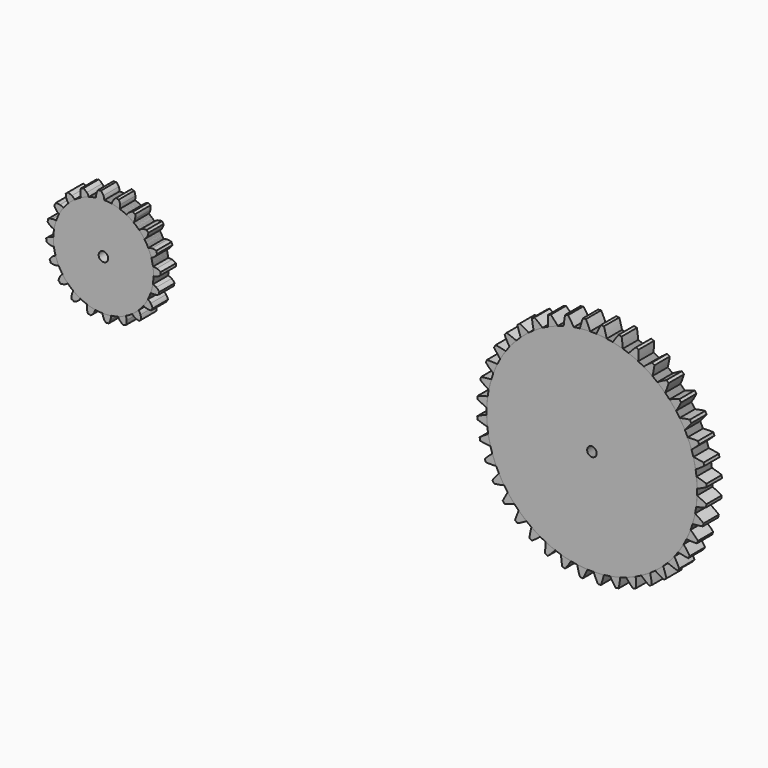
from build123d import *

# Parameters (mm, degrees)
F1_DEPTH = 25.4
F2_COUNT = 20
F4_D     = 12.7
F4_2_D   = 12.7
F4_3_D   = 12.7
F4_4_D   = 12.7
F4_5_D   = 12.7
F4_6_D   = 12.7
F4_7_D   = 12.7
F4_8_D   = 12.7
F4_9_D   = 12.7
F4_10_D  = 12.7
F4_11_D  = 12.7
F4_12_D  = 12.7
F4_13_D  = 12.7
F4_14_D  = 12.7
F4_15_D  = 12.7
F4_16_D  = 12.7
F4_17_D  = 12.7
F4_18_D  = 12.7
F4_19_D  = 12.7
F4_20_D  = 12.7
F5_R     = 6.35
F6_DEPTH = 25.4
F7_COUNT = 40


with BuildPart() as f1:
    # F0 (on Front) → F1 (new body)
    with BuildSketch(Plane.XZ):
        with BuildLine():
            ThreePointArc((-9.7867536931, 65.6960325526), (-43.3687864365, -50.3080272325), (66.421, 0))
            ThreePointArc((66.421, 0), (47.3638595406, 46.5662329421), (1.1279736855, 66.4114215807))
            ThreePointArc((1.1279736855, 66.4114215807), (-4.3441412466, 66.2787875404), (-9.7867536931, 65.6960325526))
        make_face()
        with BuildLine():
            ThreePointArc((-9.7867536931, 65.6960325526), (-4.3441412466, 66.2787875404), (1.1279736855, 66.4114215807))
            ThreePointArc((1.1279736855, 66.4114215807), (0.8169736788, 68.9502136588), (0, 71.374))
            ThreePointArc((0, 71.374), (-1.4134778135, 73.8905086139), (-3.2325792895, 76.1314023983))
            ThreePointArc((-3.2325792895, 76.1314023983), (-4.9594819457, 75.6670723933), (-6.7322179379, 75.9020239627))
            ThreePointArc((-6.7322179379, 75.9020239627), (-8.2432614157, 73.4428609463), (-9.3161764435, 70.7633855357))
            ThreePointArc((-9.3161764435, 70.7633855357), (-9.8097931974, 68.2536985592), (-9.7867536931, 65.6960325526))
        make_face()
    extrude(amount=F1_DEPTH)


with BuildPart() as f2_1:
    # F2: instance of F1
    add(f1.part.rotate(Axis((0, 0, 0), (0, 1, 0)), 1 * 360 / F2_COUNT))

    # F4#2 (through all)
    with Locations(Plane.XZ.offset(25.4)):
        with Locations((0, 0)):
            Hole(F4_2_D / 2)


with BuildPart() as f2_2:
    # F2: instance of F1
    add(f1.part.rotate(Axis((0, 0, 0), (0, 1, 0)), 2 * 360 / F2_COUNT))

    # F4#3 (through all)
    with Locations(Plane.XZ.offset(25.4)):
        with Locations((0, 0)):
            Hole(F4_3_D / 2)


with BuildPart() as f2_3:
    # F2: instance of F1
    add(f1.part.rotate(Axis((0, 0, 0), (0, 1, 0)), 3 * 360 / F2_COUNT))

    # F4#4 (through all)
    with Locations(Plane.XZ.offset(25.4)):
        with Locations((0, 0)):
            Hole(F4_4_D / 2)


with BuildPart() as f2_4:
    # F2: instance of F1
    add(f1.part.rotate(Axis((0, 0, 0), (0, 1, 0)), 4 * 360 / F2_COUNT))

    # F4#5 (through all)
    with Locations(Plane.XZ.offset(25.4)):
        with Locations((0, 0)):
            Hole(F4_5_D / 2)


with BuildPart() as f2_5:
    # F2: instance of F1
    add(f1.part.rotate(Axis((0, 0, 0), (0, 1, 0)), 5 * 360 / F2_COUNT))

    # F4#6 (through all)
    with Locations(Plane.XZ.offset(25.4)):
        with Locations((0, 0)):
            Hole(F4_6_D / 2)


with BuildPart() as f2_6:
    # F2: instance of F1
    add(f1.part.rotate(Axis((0, 0, 0), (0, 1, 0)), 6 * 360 / F2_COUNT))

    # F4#7 (through all)
    with Locations(Plane.XZ.offset(25.4)):
        with Locations((0, 0)):
            Hole(F4_7_D / 2)


with BuildPart() as f2_7:
    # F2: instance of F1
    add(f1.part.rotate(Axis((0, 0, 0), (0, 1, 0)), 7 * 360 / F2_COUNT))

    # F4#8 (through all)
    with Locations(Plane.XZ.offset(25.4)):
        with Locations((0, 0)):
            Hole(F4_8_D / 2)


with BuildPart() as f2_8:
    # F2: instance of F1
    add(f1.part.rotate(Axis((0, 0, 0), (0, 1, 0)), 8 * 360 / F2_COUNT))

    # F4#9 (through all)
    with Locations(Plane.XZ.offset(25.4)):
        with Locations((0, 0)):
            Hole(F4_9_D / 2)


with BuildPart() as f2_9:
    # F2: instance of F1
    add(f1.part.rotate(Axis((0, 0, 0), (0, 1, 0)), 9 * 360 / F2_COUNT))

    # F4#10 (through all)
    with Locations(Plane.XZ.offset(25.4)):
        with Locations((0, 0)):
            Hole(F4_10_D / 2)


with BuildPart() as f2_10:
    # F2: instance of F1
    add(f1.part.rotate(Axis((0, 0, 0), (0, 1, 0)), 10 * 360 / F2_COUNT))

    # F4#11 (through all)
    with Locations(Plane.XZ.offset(25.4)):
        with Locations((0, 0)):
            Hole(F4_11_D / 2)


with BuildPart() as f2_11:
    # F2: instance of F1
    add(f1.part.rotate(Axis((0, 0, 0), (0, 1, 0)), 11 * 360 / F2_COUNT))

    # F4#12 (through all)
    with Locations(Plane.XZ.offset(25.4)):
        with Locations((0, 0)):
            Hole(F4_12_D / 2)


with BuildPart() as f2_12:
    # F2: instance of F1
    add(f1.part.rotate(Axis((0, 0, 0), (0, 1, 0)), 12 * 360 / F2_COUNT))

    # F4#13 (through all)
    with Locations(Plane.XZ.offset(25.4)):
        with Locations((0, 0)):
            Hole(F4_13_D / 2)


with BuildPart() as f2_13:
    # F2: instance of F1
    add(f1.part.rotate(Axis((0, 0, 0), (0, 1, 0)), 13 * 360 / F2_COUNT))

    # F4#14 (through all)
    with Locations(Plane.XZ.offset(25.4)):
        with Locations((0, 0)):
            Hole(F4_14_D / 2)


with BuildPart() as f2_14:
    # F2: instance of F1
    add(f1.part.rotate(Axis((0, 0, 0), (0, 1, 0)), 14 * 360 / F2_COUNT))

    # F4#15 (through all)
    with Locations(Plane.XZ.offset(25.4)):
        with Locations((0, 0)):
            Hole(F4_15_D / 2)


with BuildPart() as f2_15:
    # F2: instance of F1
    add(f1.part.rotate(Axis((0, 0, 0), (0, 1, 0)), 15 * 360 / F2_COUNT))

    # F4#16 (through all)
    with Locations(Plane.XZ.offset(25.4)):
        with Locations((0, 0)):
            Hole(F4_16_D / 2)


with BuildPart() as f2_16:
    # F2: instance of F1
    add(f1.part.rotate(Axis((0, 0, 0), (0, 1, 0)), 16 * 360 / F2_COUNT))

    # F4#17 (through all)
    with Locations(Plane.XZ.offset(25.4)):
        with Locations((0, 0)):
            Hole(F4_17_D / 2)


with BuildPart() as f2_17:
    # F2: instance of F1
    add(f1.part.rotate(Axis((0, 0, 0), (0, 1, 0)), 17 * 360 / F2_COUNT))

    # F4#18 (through all)
    with Locations(Plane.XZ.offset(25.4)):
        with Locations((0, 0)):
            Hole(F4_18_D / 2)


with BuildPart() as f2_18:
    # F2: instance of F1
    add(f1.part.rotate(Axis((0, 0, 0), (0, 1, 0)), 18 * 360 / F2_COUNT))

    # F4#19 (through all)
    with Locations(Plane.XZ.offset(25.4)):
        with Locations((0, 0)):
            Hole(F4_19_D / 2)


with BuildPart() as f2_19:
    # F2: instance of F1
    add(f1.part.rotate(Axis((0, 0, 0), (0, 1, 0)), 19 * 360 / F2_COUNT))

    # F4#20 (through all)
    with Locations(Plane.XZ.offset(25.4)):
        with Locations((0, 0)):
            Hole(F4_20_D / 2)


with BuildPart() as f1_1:
    add(f1.part)

    # F4 (through all)
    with Locations(Plane.XZ.offset(25.4)):
        with Locations((0, 0)):
            Hole(F4_D / 2)


with BuildPart() as f6:
    # F5 (on face) → F6 (new body)
    with BuildSketch(Plane.XZ.offset(25.4)):
        with BuildLine():
            ThreePointArc((652.4994199056, 138.7851091336), (659.3245413182, 139.4008915764), (666.1716486086, 139.6812343471))
            ThreePointArc((666.1716486086, 139.6812343471), (663.4953986447, 146.021467293), (660.4418424191, 152.1888542643))
            ThreePointArc((660.4418424191, 152.1888542643), (658.501659989, 151.9556345499), (656.5476348072, 151.9336144125))
            ThreePointArc((656.5476348072, 151.9336144125), (654.3252077157, 145.4204212248), (652.4994199056, 138.7851091336))
        make_face()
        with BuildLine():
            ThreePointArc((652.4994199056, 138.7851091336), (575.4930649993, -104.2736131955), (808.1613584717, 0))
            ThreePointArc((808.1613584717, 0), (766.4312965449, 99.5890618187), (666.1716486086, 139.6812343471))
            ThreePointArc((666.1716486086, 139.6812343471), (659.3245413182, 139.4008915764), (652.4994199056, 138.7851091336))
        make_face()
        with Locations((668.4613584717, 0)):
            Circle(F5_R, mode=Mode.SUBTRACT)
    extrude(amount=F6_DEPTH)


with BuildPart() as f7_1:
    # F7: instance of F6
    add(f6.part.rotate(Axis((668.4613584717, -25.4, 0), (0, 1, 0)), 1 * 360 / F7_COUNT))


with BuildPart() as f7_2:
    # F7: instance of F6
    add(f6.part.rotate(Axis((668.4613584717, -25.4, 0), (0, 1, 0)), 2 * 360 / F7_COUNT))


with BuildPart() as f7_3:
    # F7: instance of F6
    add(f6.part.rotate(Axis((668.4613584717, -25.4, 0), (0, 1, 0)), 3 * 360 / F7_COUNT))


with BuildPart() as f7_4:
    # F7: instance of F6
    add(f6.part.rotate(Axis((668.4613584717, -25.4, 0), (0, 1, 0)), 4 * 360 / F7_COUNT))


with BuildPart() as f7_5:
    # F7: instance of F6
    add(f6.part.rotate(Axis((668.4613584717, -25.4, 0), (0, 1, 0)), 5 * 360 / F7_COUNT))


with BuildPart() as f7_6:
    # F7: instance of F6
    add(f6.part.rotate(Axis((668.4613584717, -25.4, 0), (0, 1, 0)), 6 * 360 / F7_COUNT))


with BuildPart() as f7_7:
    # F7: instance of F6
    add(f6.part.rotate(Axis((668.4613584717, -25.4, 0), (0, 1, 0)), 7 * 360 / F7_COUNT))


with BuildPart() as f7_8:
    # F7: instance of F6
    add(f6.part.rotate(Axis((668.4613584717, -25.4, 0), (0, 1, 0)), 8 * 360 / F7_COUNT))


with BuildPart() as f7_9:
    # F7: instance of F6
    add(f6.part.rotate(Axis((668.4613584717, -25.4, 0), (0, 1, 0)), 9 * 360 / F7_COUNT))


with BuildPart() as f7_10:
    # F7: instance of F6
    add(f6.part.rotate(Axis((668.4613584717, -25.4, 0), (0, 1, 0)), 10 * 360 / F7_COUNT))


with BuildPart() as f7_11:
    # F7: instance of F6
    add(f6.part.rotate(Axis((668.4613584717, -25.4, 0), (0, 1, 0)), 11 * 360 / F7_COUNT))


with BuildPart() as f7_12:
    # F7: instance of F6
    add(f6.part.rotate(Axis((668.4613584717, -25.4, 0), (0, 1, 0)), 12 * 360 / F7_COUNT))


with BuildPart() as f7_13:
    # F7: instance of F6
    add(f6.part.rotate(Axis((668.4613584717, -25.4, 0), (0, 1, 0)), 13 * 360 / F7_COUNT))


with BuildPart() as f7_14:
    # F7: instance of F6
    add(f6.part.rotate(Axis((668.4613584717, -25.4, 0), (0, 1, 0)), 14 * 360 / F7_COUNT))


with BuildPart() as f7_15:
    # F7: instance of F6
    add(f6.part.rotate(Axis((668.4613584717, -25.4, 0), (0, 1, 0)), 15 * 360 / F7_COUNT))


with BuildPart() as f7_16:
    # F7: instance of F6
    add(f6.part.rotate(Axis((668.4613584717, -25.4, 0), (0, 1, 0)), 16 * 360 / F7_COUNT))


with BuildPart() as f7_17:
    # F7: instance of F6
    add(f6.part.rotate(Axis((668.4613584717, -25.4, 0), (0, 1, 0)), 17 * 360 / F7_COUNT))


with BuildPart() as f7_18:
    # F7: instance of F6
    add(f6.part.rotate(Axis((668.4613584717, -25.4, 0), (0, 1, 0)), 18 * 360 / F7_COUNT))


with BuildPart() as f7_19:
    # F7: instance of F6
    add(f6.part.rotate(Axis((668.4613584717, -25.4, 0), (0, 1, 0)), 19 * 360 / F7_COUNT))


with BuildPart() as f7_20:
    # F7: instance of F6
    add(f6.part.rotate(Axis((668.4613584717, -25.4, 0), (0, 1, 0)), 20 * 360 / F7_COUNT))


with BuildPart() as f7_21:
    # F7: instance of F6
    add(f6.part.rotate(Axis((668.4613584717, -25.4, 0), (0, 1, 0)), 21 * 360 / F7_COUNT))


with BuildPart() as f7_22:
    # F7: instance of F6
    add(f6.part.rotate(Axis((668.4613584717, -25.4, 0), (0, 1, 0)), 22 * 360 / F7_COUNT))


with BuildPart() as f7_23:
    # F7: instance of F6
    add(f6.part.rotate(Axis((668.4613584717, -25.4, 0), (0, 1, 0)), 23 * 360 / F7_COUNT))


with BuildPart() as f7_24:
    # F7: instance of F6
    add(f6.part.rotate(Axis((668.4613584717, -25.4, 0), (0, 1, 0)), 24 * 360 / F7_COUNT))


with BuildPart() as f7_25:
    # F7: instance of F6
    add(f6.part.rotate(Axis((668.4613584717, -25.4, 0), (0, 1, 0)), 25 * 360 / F7_COUNT))


with BuildPart() as f7_26:
    # F7: instance of F6
    add(f6.part.rotate(Axis((668.4613584717, -25.4, 0), (0, 1, 0)), 26 * 360 / F7_COUNT))


with BuildPart() as f7_27:
    # F7: instance of F6
    add(f6.part.rotate(Axis((668.4613584717, -25.4, 0), (0, 1, 0)), 27 * 360 / F7_COUNT))


with BuildPart() as f7_28:
    # F7: instance of F6
    add(f6.part.rotate(Axis((668.4613584717, -25.4, 0), (0, 1, 0)), 28 * 360 / F7_COUNT))


with BuildPart() as f7_29:
    # F7: instance of F6
    add(f6.part.rotate(Axis((668.4613584717, -25.4, 0), (0, 1, 0)), 29 * 360 / F7_COUNT))


with BuildPart() as f7_30:
    # F7: instance of F6
    add(f6.part.rotate(Axis((668.4613584717, -25.4, 0), (0, 1, 0)), 30 * 360 / F7_COUNT))


with BuildPart() as f7_31:
    # F7: instance of F6
    add(f6.part.rotate(Axis((668.4613584717, -25.4, 0), (0, 1, 0)), 31 * 360 / F7_COUNT))


with BuildPart() as f7_32:
    # F7: instance of F6
    add(f6.part.rotate(Axis((668.4613584717, -25.4, 0), (0, 1, 0)), 32 * 360 / F7_COUNT))


with BuildPart() as f7_33:
    # F7: instance of F6
    add(f6.part.rotate(Axis((668.4613584717, -25.4, 0), (0, 1, 0)), 33 * 360 / F7_COUNT))


with BuildPart() as f7_34:
    # F7: instance of F6
    add(f6.part.rotate(Axis((668.4613584717, -25.4, 0), (0, 1, 0)), 34 * 360 / F7_COUNT))


with BuildPart() as f7_35:
    # F7: instance of F6
    add(f6.part.rotate(Axis((668.4613584717, -25.4, 0), (0, 1, 0)), 35 * 360 / F7_COUNT))


with BuildPart() as f7_36:
    # F7: instance of F6
    add(f6.part.rotate(Axis((668.4613584717, -25.4, 0), (0, 1, 0)), 36 * 360 / F7_COUNT))


with BuildPart() as f7_37:
    # F7: instance of F6
    add(f6.part.rotate(Axis((668.4613584717, -25.4, 0), (0, 1, 0)), 37 * 360 / F7_COUNT))


with BuildPart() as f7_38:
    # F7: instance of F6
    add(f6.part.rotate(Axis((668.4613584717, -25.4, 0), (0, 1, 0)), 38 * 360 / F7_COUNT))


with BuildPart() as f7_39:
    # F7: instance of F6
    add(f6.part.rotate(Axis((668.4613584717, -25.4, 0), (0, 1, 0)), 39 * 360 / F7_COUNT))


solid = Compound([f2_1.part, f2_2.part, f2_3.part, f2_4.part, f2_5.part, f2_6.part, f2_7.part, f2_8.part, f2_9.part, f2_10.part, f2_11.part, f2_12.part, f2_13.part, f2_14.part, f2_15.part, f2_16.part, f2_17.part, f2_18.part, f2_19.part, f1_1.part, f6.part, f7_1.part, f7_2.part, f7_3.part, f7_4.part, f7_5.part, f7_6.part, f7_7.part, f7_8.part, f7_9.part, f7_10.part, f7_11.part, f7_12.part, f7_13.part, f7_14.part, f7_15.part, f7_16.part, f7_17.part, f7_18.part, f7_19.part, f7_20.part, f7_21.part, f7_22.part, f7_23.part, f7_24.part, f7_25.part, f7_26.part, f7_27.part, f7_28.part, f7_29.part, f7_30.part, f7_31.part, f7_32.part, f7_33.part, f7_34.part, f7_35.part, f7_36.part, f7_37.part, f7_38.part, f7_39.part])
